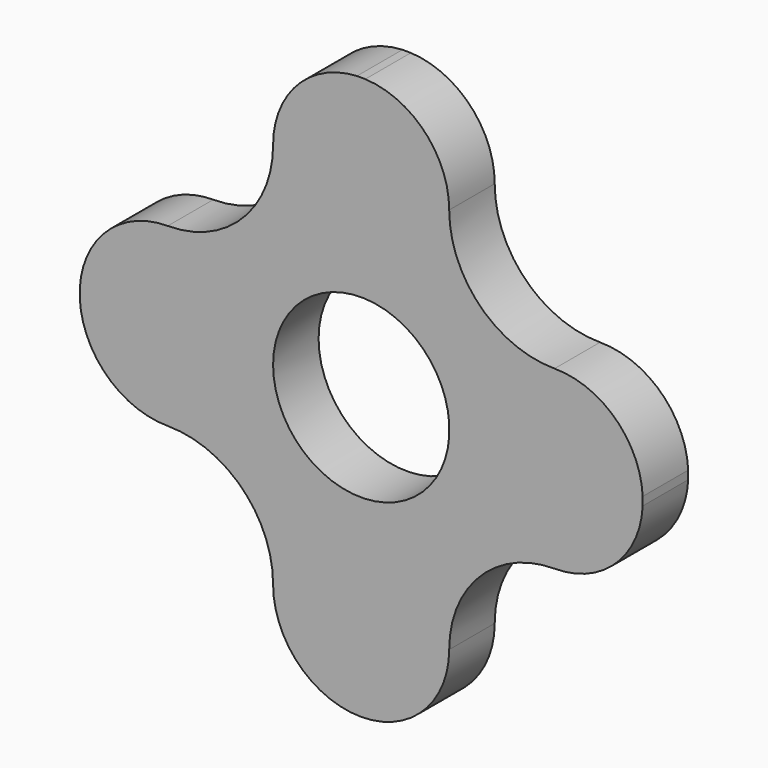
from build123d import *

# Parameters (mm, degrees)
F0_R      = 35.56
F1_DEPTH  = 7.1882
F2_R      = 11.1379
F3_DEPTH  = 7.62
F7_DEPTH  = 7.1882
F9_DEPTH  = 7.1882
F11_DEPTH = 7.1882
F13_DEPTH = 7.1882
F15_DEPTH = 25.4


# Not quite as in the source:
# - a feature of the source that left no trace in its solid (it failed there, or was rolled back) is left out


with BuildPart() as f1:
    # F0 (on Front) → F1 (new body)
    with BuildSketch(Plane.XZ):
        Circle(F0_R)
    extrude(amount=F1_DEPTH)

    # F2 (on face) → F3 (cut)
    with BuildSketch(Plane(origin=(0, 0, 0), x_dir=(-1, 0, 0), z_dir=(0, 1, 0))):
        Circle(F2_R)
    extrude(amount=-F3_DEPTH, mode=Mode.SUBTRACT)

    # F6 (on face) → F7 (join)
    with BuildSketch(Plane.XZ.offset(7.1882)):
        with BuildLine():
            Line((35.56, 11.1379), (33.7707089589, 11.1379))
            ThreePointArc((33.7707089589, 11.1379), (35.1098277593, 5.6403541298), (35.56, 0))
            Line((35.56, 0), (35.56, 11.1379))
        make_face()
        with BuildLine():
            Line((35.56, -11.1125), (35.56, 0))
            ThreePointArc((35.56, 0), (35.1119461572, -5.6271517709), (33.7790755313, -11.1125))
            Line((33.7790755313, -11.1125), (35.56, -11.1125))
        make_face()
    extrude(amount=-F7_DEPTH)

    # F8 (on face) → F9 (join)
    with BuildSketch(Plane.XZ.offset(7.1882)):
        with BuildLine():
            Line((-11.1379, 35.56), (-11.1379, 33.7707089589))
            ThreePointArc((-11.1379, 33.7707089589), (-5.6403540801, 35.1098277673), (1.006e-07, 35.56))
            Line((1.006e-07, 35.56), (-11.1379, 35.56))
        make_face()
        with BuildLine():
            Line((11.1125, 35.56), (1.006e-07, 35.56))
            ThreePointArc((1.006e-07, 35.56), (5.6271518206, 35.1119461492), (11.1125, 33.7790755313))
            Line((11.1125, 33.7790755313), (11.1125, 35.56))
        make_face()
    extrude(amount=-F9_DEPTH)

    # F10 (on face) → F11 (join)
    with BuildSketch(Plane.XZ.offset(7.1882)):
        with BuildLine():
            ThreePointArc((-35.56, 0), (-35.1119461572, 5.627151771), (-33.7790755313, 11.1125))
            Line((-33.7790755313, 11.1125), (-35.56, 11.1125))
            Line((-35.56, 11.1125), (-35.56, 0))
        make_face()
        with BuildLine():
            Line((-35.56, -11.1379), (-33.7707089589, -11.1379))
            ThreePointArc((-33.7707089589, -11.1379), (-35.1098277593, -5.6403541298), (-35.56, 0))
            Line((-35.56, 0), (-35.56, -11.1379))
        make_face()
    extrude(amount=-F11_DEPTH)

    # F12 (on face) → F13 (join)
    with BuildSketch(Plane.XZ.offset(7.1882)):
        with BuildLine():
            ThreePointArc((0, -35.56), (-5.6403541298, -35.1098277593), (-11.1379, -33.7707089589))
            Line((-11.1379, -33.7707089589), (-11.1379, -35.56))
            Line((-11.1379, -35.56), (0, -35.56))
        make_face()
        with BuildLine():
            Line((11.1125, -35.56), (11.1125, -33.7790755313))
            ThreePointArc((11.1125, -33.7790755313), (5.6271517709, -35.1119461572), (0, -35.56))
            Line((0, -35.56), (11.1125, -35.56))
        make_face()
    extrude(amount=-F13_DEPTH)

    # F14 (on face) → F15 (cut)
    with BuildSketch(Plane.XZ.offset(7.1882)):
        with BuildLine():
            ThreePointArc((-11.1379, 24.4221), (-8.0739891454, 32.1147190965), (-0.5444488019, 35.56))
            Line((-0.5444488019, 35.56), (-11.1379, 35.56))
            Line((-11.1379, 35.56), (-11.1379, 33.7707089589))
            ThreePointArc((-11.1379, 33.7707089589), (-25.1541702512, 25.1352604716), (-33.7790755313, 11.1125))
            Line((-33.7790755313, 11.1125), (-35.56, 11.1125))
            Line((-35.56, 11.1125), (-35.56, 0.5190198064))
            ThreePointArc((-35.56, 0.5190198064), (-32.1239164631, 8.03980237), (-24.4475, 11.1125))
            ThreePointArc((-24.4475, 11.1125), (-15.0361915851, 15.0107915851), (-11.1379, 24.4221))
        make_face()
        with BuildLine():
            Line((-0.5444488019, 35.56), (0.5190198064, 35.56))
            ThreePointArc((0.5190198064, 35.56), (-0.0127144977, 35.5727144977), (-0.5444488019, 35.56))
        make_face()
        with BuildLine():
            ThreePointArc((0.5190198064, 35.56), (8.03980237, 32.1239164631), (11.1125, 24.4475))
            ThreePointArc((11.1125, 24.4475), (15.0107915851, 15.0361915851), (24.4221, 11.1379))
            ThreePointArc((24.4221, 11.1379), (32.1147190965, 8.0739891454), (35.56, 0.5444488019))
            Line((35.56, 0.5444488019), (35.56, 11.1379))
            Line((35.56, 11.1379), (33.7707089589, 11.1379))
            ThreePointArc((33.7707089589, 11.1379), (25.1352604716, 25.1541702512), (11.1125, 33.7790755313))
            Line((11.1125, 33.7790755313), (11.1125, 35.56))
            Line((11.1125, 35.56), (0.5190198064, 35.56))
        make_face()
        with BuildLine():
            ThreePointArc((35.56, -0.5190198064), (35.5727144977, 0.0127144977), (35.56, 0.5444488019))
            Line((35.56, 0.5444488019), (35.56, -0.5190198064))
        make_face()
        with BuildLine():
            Line((35.56, -11.1125), (35.56, -0.5190198064))
            ThreePointArc((35.56, -0.5190198064), (32.1239164631, -8.03980237), (24.4475, -11.1125))
            ThreePointArc((24.4475, -11.1125), (15.0182310729, -15.0182310729), (11.1125, -24.4475))
            ThreePointArc((11.1125, -24.4475), (-0.0253855106, -35.5473072489), (-11.1379, -24.4221))
            ThreePointArc((-11.1379, -24.4221), (-15.0287520974, -15.0287520974), (-24.4221, -11.1379))
            ThreePointArc((-24.4221, -11.1379), (-32.1147190965, -8.0739891454), (-35.56, -0.5444488019))
            Line((-35.56, -0.5444488019), (-35.56, -11.1379))
            Line((-35.56, -11.1379), (-33.7707089589, -11.1379))
            ThreePointArc((-33.7707089589, -11.1379), (-25.144717139, -25.144717139), (-11.1379, -33.7707089589))
            Line((-11.1379, -33.7707089589), (-11.1379, -35.56))
            Line((-11.1379, -35.56), (11.1125, -35.56))
            Line((11.1125, -35.56), (11.1125, -33.7790755313))
            ThreePointArc((11.1125, -33.7790755313), (25.144717139, -25.144717139), (33.7790755313, -11.1125))
            Line((33.7790755313, -11.1125), (35.56, -11.1125))
        make_face()
        with BuildLine():
            Line((-35.56, -0.5444488019), (-35.56, 0.5190198064))
            ThreePointArc((-35.56, 0.5190198064), (-35.5727144977, -0.0127144977), (-35.56, -0.5444488019))
        make_face()
    extrude(amount=-F15_DEPTH, mode=Mode.SUBTRACT)


solid = f1.part
